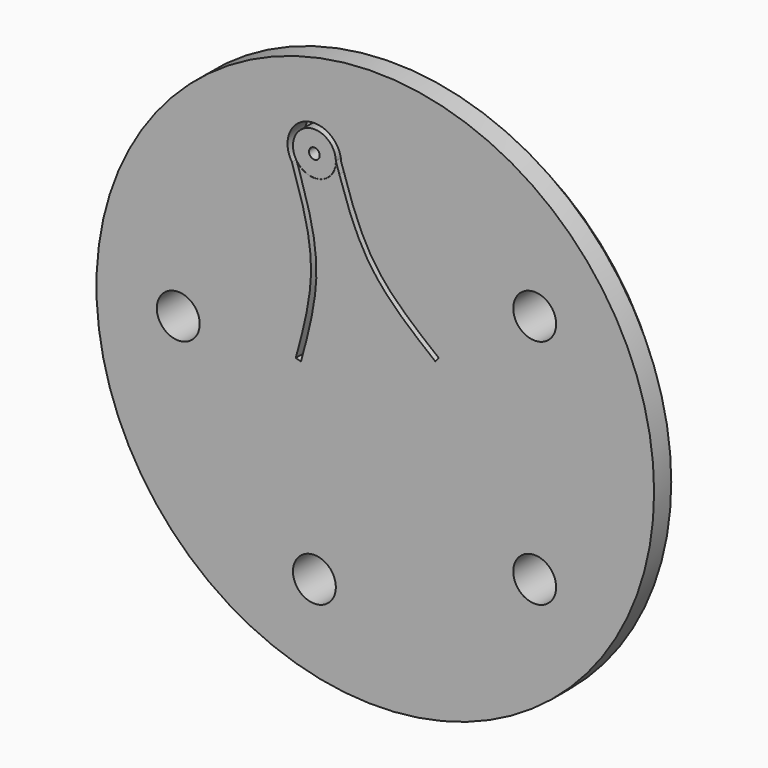
from build123d import *

# Parameters (mm, degrees)
F0_R     = 76.2
F0_R_2   = 6.35
F0_R_3   = 9.525
F1_DEPTH = 6.35
F2_R     = 82.55
F2_R_2   = 76.2
F2_R_3   = 6.35
F3_DEPTH = 6.35


# Not quite as in the source:
# - a length typed as a fraction of an inch, garbled in the dataset ("3 / 203.2 mm" for 3/8 in), is restored
# - the dataset's text gives a spline's control points without its knots; the knots are read off the source's solid


with BuildPart() as f1:
    # F0 (on Front) → F1 (new body)
    with BuildSketch(Plane.XZ):
        Circle(F0_R)
        with Locations((-18.0268847294, -55.4810463583)):
            Circle(F0_R_2, mode=Mode.SUBTRACT)
        with Locations((-47.1949969329, -34.2891723808)):
            Circle(F0_R_2, mode=Mode.SUBTRACT)
        with Locations((18.0268847294, -55.4810463583)):
            Circle(F0_R_2, mode=Mode.SUBTRACT)
        with Locations((47.1949969329, -34.2891723808)):
            Circle(F0_R_2, mode=Mode.SUBTRACT)
        with Locations((-58.336224407, 0)):
            Circle(F0_R_2, mode=Mode.SUBTRACT)
        with Locations((-47.1949969329, 34.2891723808)):
            Circle(F0_R_2, mode=Mode.SUBTRACT)
        with Locations((-18.0268847294, 55.4810463583)):
            Circle(F0_R_2, mode=Mode.SUBTRACT)
        Circle(F0_R_3, mode=Mode.SUBTRACT)
        with Locations((58.336224407, 0)):
            Circle(F0_R_2, mode=Mode.SUBTRACT)
        with Locations((47.1949969329, 34.2891723808)):
            Circle(F0_R_2, mode=Mode.SUBTRACT)
        with Locations((18.0268847294, 55.4810463583)):
            Circle(F0_R_2, mode=Mode.SUBTRACT)
    extrude(amount=F1_DEPTH)

    # F2 (on face) → F3 (join)
    with BuildSketch(Plane.XZ.offset(6.35)):
        Circle(F2_R)
        Circle(F2_R_2, mode=Mode.SUBTRACT)
        Circle(F2_R_2)
        with Locations((-18.0268847294, -55.4810463583)):
            Circle(F2_R_3, mode=Mode.SUBTRACT)
        with Locations((-47.1949969329, -34.2891723808)):
            Circle(F2_R_3, mode=Mode.SUBTRACT)
        with Locations((18.0268847294, -55.4810463583)):
            Circle(F2_R_3, mode=Mode.SUBTRACT)
        with Locations((47.1949969329, -34.2891723808)):
            Circle(F2_R_3, mode=Mode.SUBTRACT)
        with Locations((-58.336224407, 0)):
            Circle(F2_R_3, mode=Mode.SUBTRACT)
        with Locations((-47.1949969329, 34.2891723808)):
            Circle(F2_R_3, mode=Mode.SUBTRACT)
        with BuildLine():
            add(Edge.make_bspline(
                [(-10.6542657196, 52.4734320289), (-8.2332526855, 45.0247226448), (-2.5822173462, 29.3020077299), (10.6983686228, 18.6386544846), (17.8031913761, 12.934775669)],
                knots=[0.0620717582, 0.0620717582, 0.0620717582, 0.0620717582, 0.4982746672, 1, 1, 1, 1], degree=3))
            ThreePointArc((-10.6542657196, 52.4734320289), (-12.6062796926, 49.6485258008), (-15.5663398463, 47.908267879))
            ThreePointArc((-15.5663398463, 47.908267879), (-18.9839767566, 47.5762864081), (-22.223627454, 48.7143185285))
            add(Edge.make_bspline(
                [(-22.223627454, 48.7143185285), (-19.8040266177, 41.2651502936), (-15.13423029, 25.2236114971), (-19.6106882565, 8.7906449303), (-22.0059547573, 0)],
                knots=[0.0620717582, 0.0620717582, 0.0620717582, 0.0620717582, 0.4982746672, 1, 1, 1, 1], degree=3))
            Line((-22.0059547573, 0), (-23.5376137966, 0.4173449862))
            add(Edge.make_bspline(
                [(-24.6771337574, 51.1020689794), (-24.0063692851, 49.0670118083), (-22.6416674455, 44.9146579119), (-20.8291476072, 38.6791660774), (-19.7093838867, 33.4359520654), (-19.1757596195, 29.2572537264), (-18.9844511798, 26.1346205763), (-19.0278027605, 23.000080355), (-19.360603347, 18.7820552575), (-20.2248090599, 13.4503695291), (-21.7522886479, 6.9703254819), (-22.940861019, 2.6074318834), (-23.5376137966, 0.4173449862)],
                knots=[0.0057570398, 0.0057570398, 0.0057570398, 0.0057570398, 0.125, 0.25, 0.375, 0.4375, 0.5, 0.5625, 0.625, 0.75, 0.875, 1, 1, 1, 1], degree=3))
            ThreePointArc((-24.6771337574, 51.1020689794), (-20.4874296126, 63.0538248376), (-10.0728219256, 55.8472975435))
            add(Edge.make_bspline(
                [(-10.0728219256, 55.8472975435), (-9.4193051901, 53.806636243), (-8.0826797879, 49.645159759), (-5.8839089986, 43.5351684662), (-3.7079330074, 38.6351386244), (-1.6834668507, 34.9408441793), (-0.0028009157, 32.3021326141), (1.8747077646, 29.7917177253), (4.623242041, 26.5748790154), (8.4562853904, 22.7694220255), (13.5009166607, 18.424786242), (17.0269364225, 15.5937564872), (18.7970203404, 14.1727014502)],
                knots=[0.0057570398, 0.0057570398, 0.0057570398, 0.0057570398, 0.125, 0.25, 0.375, 0.4375, 0.5, 0.5625, 0.625, 0.75, 0.875, 1, 1, 1, 1], degree=3))
            Line((18.7970203404, 14.1727014502), (17.8031913761, 12.934775669))
        make_face(mode=Mode.SUBTRACT)
        with BuildLine():
            ThreePointArc((9.525, 0), (-5.5986545281, -7.7058868714), (-2.9433868714, 9.0588133177))
            ThreePointArc((-2.9433868714, 9.0588133177), (5.5986545281, 7.7058868714), (9.525, 0))
        make_face(mode=Mode.SUBTRACT)
        with Locations((58.336224407, 0)):
            Circle(F2_R_3, mode=Mode.SUBTRACT)
        with Locations((47.1949969329, 34.2891723808)):
            Circle(F2_R_3, mode=Mode.SUBTRACT)
        with Locations((18.0268847294, 55.4810463583)):
            Circle(F2_R_3, mode=Mode.SUBTRACT)
        with BuildLine():
            ThreePointArc((9.525, 0), (5.5986545281, 7.7058868714), (-2.9433868714, 9.0588133177))
            ThreePointArc((-2.9433868714, 9.0588133177), (-5.5986545281, -7.7058868714), (9.525, 0))
        make_face()
        with BuildLine():
            ThreePointArc((6.35, 0), (-3.7324363521, -5.1372579143), (-1.9622579143, 6.0392088785))
            ThreePointArc((-1.9622579143, 6.0392088785), (3.7324363521, 5.1372579143), (6.35, 0))
        make_face(mode=Mode.SUBTRACT)
        with BuildLine():
            ThreePointArc((-11.6768847294, 55.4810463583), (-11.6775070317, 55.5699443457), (-11.6793738167, 55.6588249089))
            ThreePointArc((-11.6793738167, 55.6588249089), (-19.9891426437, 61.5202552368), (-23.26662454, 51.8938989238))
            ThreePointArc((-23.26662454, 51.8938989238), (-20.0734973519, 49.4699003134), (-16.0646268151, 49.4418374798))
            ThreePointArc((-16.0646268151, 49.4418374798), (-12.8896268151, 51.7486100062), (-11.6768847294, 55.4810463583))
        make_face()
        with BuildLine():
            ThreePointArc((-16.4393847294, 55.4810463583), (-16.7425702509, 54.5479372703), (-17.5363202509, 53.9712441387))
            ThreePointArc((-17.5363202509, 53.9712441387), (-19.311199208, 56.4141554463), (-16.4393847294, 55.4810463583))
        make_face(mode=Mode.SUBTRACT)
        with BuildLine():
            ThreePointArc((6.35, 0), (3.7324363521, 5.1372579143), (-1.9622579143, 6.0392088785))
            ThreePointArc((-1.9622579143, 6.0392088785), (-3.7324363521, -5.1372579143), (6.35, 0))
        make_face()
        with Locations((-47.1949969329, -34.2891723808)):
            Circle(F2_R_3)
        with Locations((18.0268847294, -55.4810463583)):
            Circle(F2_R_3)
        with Locations((-47.1949969329, 34.2891723808)):
            Circle(F2_R_3)
        with Locations((58.336224407, 0)):
            Circle(F2_R_3)
        with Locations((18.0268847294, 55.4810463583)):
            Circle(F2_R_3)
        with BuildLine():
            ThreePointArc((-11.6525891829, 55.5751750194), (-11.6520679675, 55.5281119716), (-11.6518942259, 55.4810463583))
            ThreePointArc((-11.6518942259, 55.4810463583), (-12.8694090731, 51.7339209568), (-16.0569043249, 49.4180700986))
            Line((-16.0569043249, 49.4180700986), (-15.5663398463, 47.908267879))
            ThreePointArc((-15.5663398463, 47.908267879), (-12.6062796926, 49.6485258008), (-10.6542657196, 52.4734320289))
            add(Edge.make_bspline(
                [(-11.6525891829, 55.5751750194), (-11.3212318788, 54.5403378936), (-10.9897372013, 53.5055741688), (-10.6542657196, 52.4734320289)],
                knots=[0.0016286156, 0.0016286156, 0.0016286156, 0.0016286156, 0.0620717582, 0.0620717582, 0.0620717582, 0.0620717582], degree=3))
        make_face()
        with BuildLine():
            Line((-15.5663398463, 47.908267879), (-16.0569043249, 49.4180700986))
            ThreePointArc((-16.0569043249, 49.4180700986), (-20.0415735031, 49.4327794111), (-23.2391255926, 51.8104811288))
            add(Edge.make_bspline(
                [(-23.2391255926, 51.8104811288), (-22.8989372817, 50.778513371), (-22.5589032523, 49.7465242498), (-22.223627454, 48.7143185285)],
                knots=[0.0016286156, 0.0016286156, 0.0016286156, 0.0016286156, 0.0620717582, 0.0620717582, 0.0620717582, 0.0620717582], degree=3))
            ThreePointArc((-22.223627454, 48.7143185285), (-18.9839767566, 47.5762864081), (-15.5663398463, 47.908267879))
        make_face()
    extrude(amount=F3_DEPTH)


solid = f1.part
